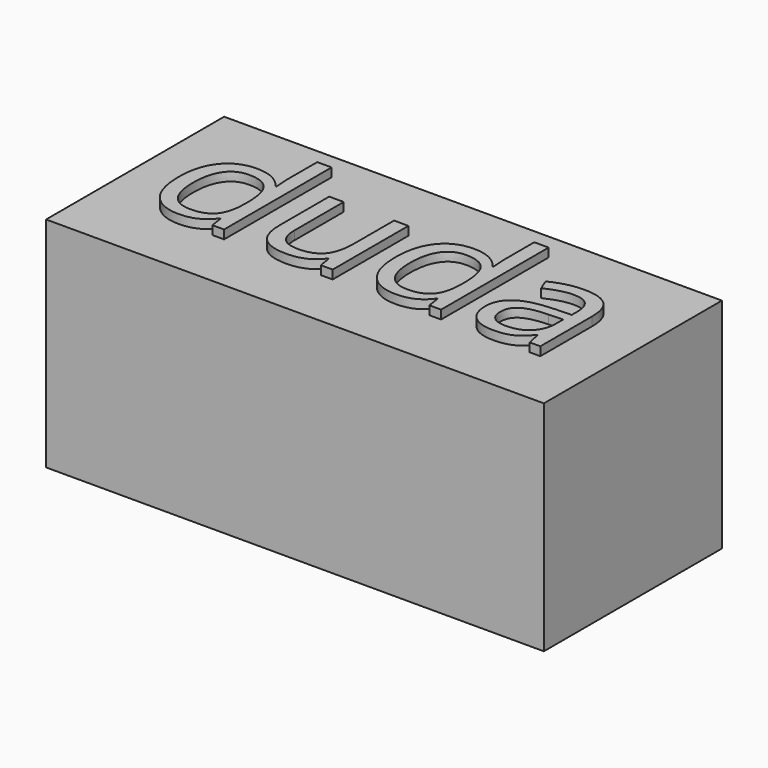
from build123d import *

# Parameters (mm, degrees)
F0_W         = 57.0065435022
F0_H         = 25.4893312231
F1_DEPTH     = 25
F2_TEXT_SIZE = 20.2605702824
F3_DEPTH     = 1


# Not quite as in the source:
# - Text() gives the source's letters only with a copy of the font that has no kerning and outlines rounded to 1/6400 em; it was checked with that copy


with BuildPart() as f1:
    # F0 (on Top) → F1 (new body)
    with BuildSketch(Plane.XY):
        with Locations((2.8328569606, -2.1954732947)):
            Rectangle(F0_W, F0_H)
    extrude(amount=F1_DEPTH)

    # F2 (on face) → F3 (join)
    with BuildSketch(Plane.XY.offset(25)):
        with Locations((-21.5052030981, -8.0106452187)):
            Text('duda', F2_TEXT_SIZE, font='Open Sans', text_align=(TextAlign.LEFT, TextAlign.BOTTOM))
    extrude(amount=F3_DEPTH)


solid = f1.part
